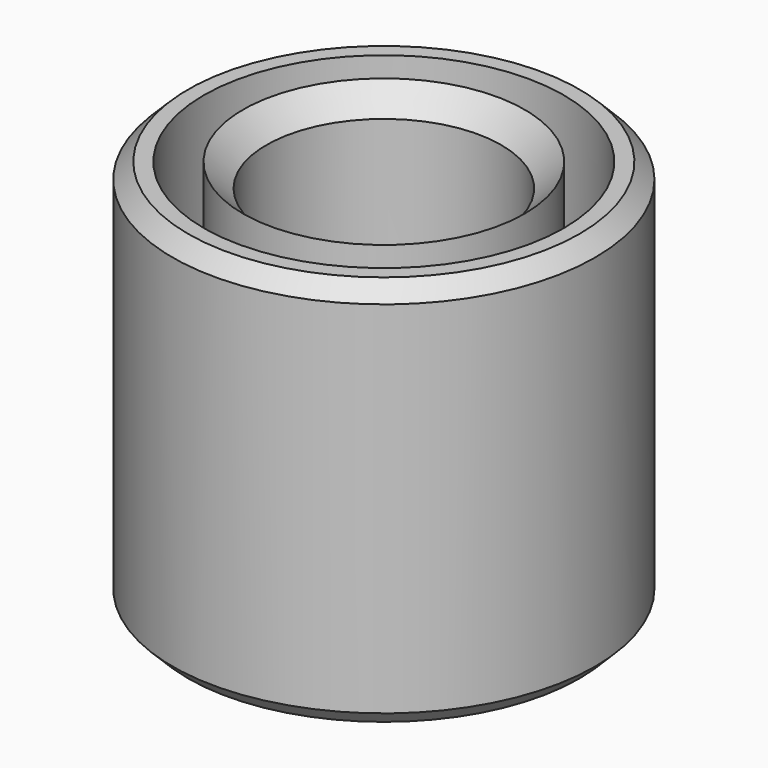
from build123d import *

# Parameters (mm, degrees)
F2_R     = 13.5
F2_R_2   = 11.5
F2_R_3   = 9
F2_R_4   = 7.5
F3_DEPTH = 2
F4_DEPTH = 25
F5_SIZE  = 1.49999
F6_SIZE  = 1


# Not quite as in the source:
# - a fillet or chamfer is up to 0.001 mm smaller than in the source, because OpenCascade refuses the exact size


with BuildPart() as f3:
    # F2 (on Top) → F3 (new body)
    with BuildSketch(Plane.XY):
        Circle(F2_R)
        Circle(F2_R_2, mode=Mode.SUBTRACT)
        Circle(F2_R_2)
        Circle(F2_R_3, mode=Mode.SUBTRACT)
        Circle(F2_R_3)
        Circle(F2_R_4, mode=Mode.SUBTRACT)
    extrude(amount=F3_DEPTH)

    # F2 (on Top) → F4 (join)
    with BuildSketch(Plane.XY):
        Circle(F2_R)
        Circle(F2_R_2, mode=Mode.SUBTRACT)
        Circle(F2_R_3)
        Circle(F2_R_4, mode=Mode.SUBTRACT)
    extrude(amount=F4_DEPTH)

    # F5 (size 1.5 in the source; OpenCascade refuses exactly that, so slightly less here)
    f5_edges = [f3.edges().sort_by_distance(p)[0] for p in [
        (-7.5, 0, 25),
    ]]
    chamfer(f5_edges, length=F5_SIZE)

    # F6
    f6_edges = [f3.edges().sort_by_distance(p)[0] for p in [
        (-13.5, 0, 25),
        (-13.5, 0, 0),
        (-7.5, 0, 0),
    ]]
    chamfer(f6_edges, length=F6_SIZE)


solid = f3.part
